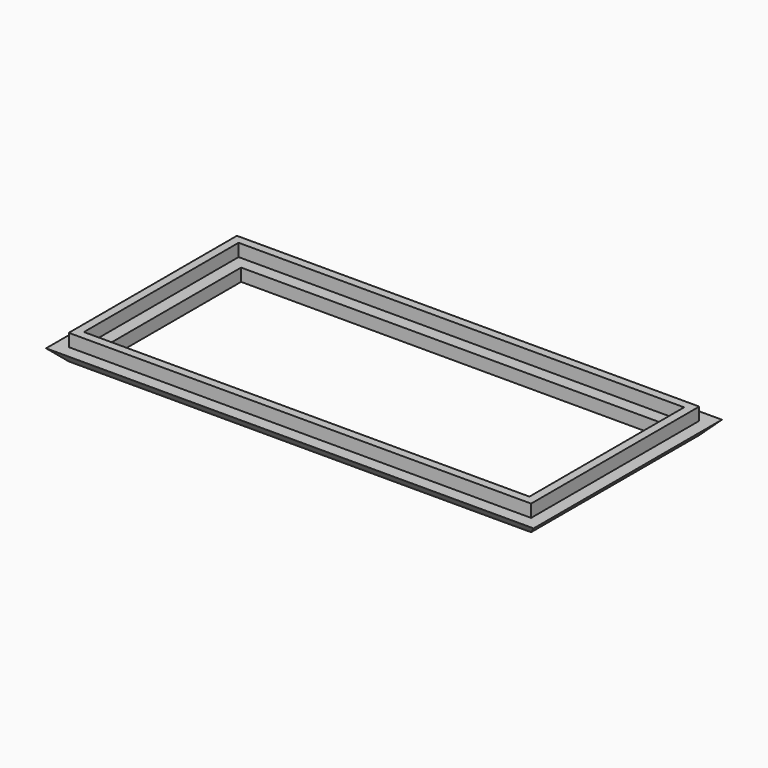
from build123d import *

# Parameters (mm, degrees)
F0_W     = 58
F0_H     = 28
F0_W_2   = 55
F0_H_2   = 25
F0_W_3   = 53
F0_H_3   = 23
F0_W_4   = 50
F0_H_4   = 20
F1_DEPTH = 1.5
F2_DEPTH = 1.5
F3_SIZE  = 1.49999


# Not quite as in the source:
# - a fillet or chamfer is up to 0.001 mm smaller than in the source, because OpenCascade refuses the exact size


with BuildPart() as f1:
    # F0 (on Top) → F1 (new body)
    with BuildSketch(Plane.XY):
        Rectangle(F0_W, F0_H)
        Rectangle(F0_W_2, F0_H_2, mode=Mode.SUBTRACT)
        Rectangle(F0_W_2, F0_H_2)
        Rectangle(F0_W_3, F0_H_3, mode=Mode.SUBTRACT)
        Rectangle(F0_W_3, F0_H_3)
        Rectangle(F0_W_4, F0_H_4, mode=Mode.SUBTRACT)
    extrude(amount=-F1_DEPTH)

    # F0 (on Top) → F2 (join)
    with BuildSketch(Plane.XY):
        Rectangle(F0_W_2, F0_H_2)
        Rectangle(F0_W_3, F0_H_3, mode=Mode.SUBTRACT)
    extrude(amount=F2_DEPTH)

    # F3 (size 1.5 in the source; OpenCascade refuses exactly that, so slightly less here)
    f3_edges = [f1.edges().sort_by_distance(p)[0] for p in [
        (0, -14, -1.5),
        (-29, 0, -1.5),
        (0, 14, -1.5),
        (29, 0, -1.5),
    ]]
    chamfer(f3_edges, length=F3_SIZE)


solid = f1.part
